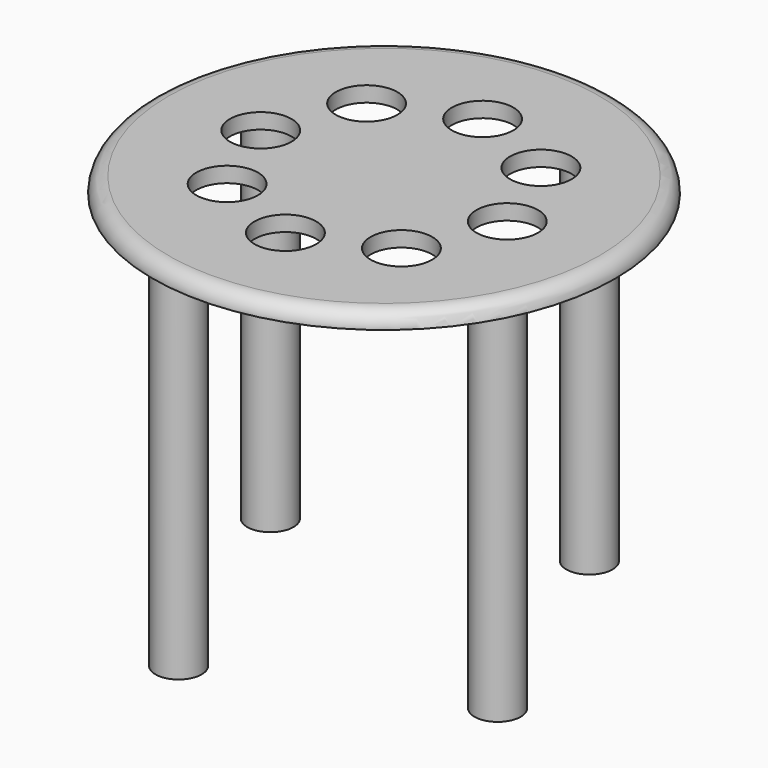
from build123d import *

# Parameters (mm, degrees)
F0_R     = 75
F0_R_2   = 10
F1_DEPTH = 5
F2_R     = 4.99999
F3_R     = 7.5
F4_DEPTH = 120


# Not quite as in the source:
# - a fillet or chamfer is up to 0.001 mm smaller than in the source, because OpenCascade refuses the exact size


with BuildPart() as f1:
    # F0 (on Top) → F1 (new body)
    with BuildSketch(Plane.XY):
        Circle(F0_R)
        with Locations((-28.2842712475, -28.2842712475)):
            Circle(F0_R_2, mode=Mode.SUBTRACT)
        with Locations((0, -40)):
            Circle(F0_R_2, mode=Mode.SUBTRACT)
        with Locations((28.2842712475, -28.2842712475)):
            Circle(F0_R_2, mode=Mode.SUBTRACT)
        with Locations((-40, 0)):
            Circle(F0_R_2, mode=Mode.SUBTRACT)
        with Locations((-28.2842712475, 28.2842712475)):
            Circle(F0_R_2, mode=Mode.SUBTRACT)
        with Locations((28.2842712475, 28.2842712475)):
            Circle(F0_R_2, mode=Mode.SUBTRACT)
        with Locations((40, 0)):
            Circle(F0_R_2, mode=Mode.SUBTRACT)
        with Locations((0, 40)):
            Circle(F0_R_2, mode=Mode.SUBTRACT)
    extrude(amount=F1_DEPTH)

    # F2 (radius 5 in the source; OpenCascade refuses exactly that, so slightly less here)
    f2_edges = [f1.edges().sort_by_distance(p)[0] for p in [
        (-75, 0, 5),
    ]]
    fillet(f2_edges, radius=F2_R)

    # F3 (on face) → F4 (join)
    with BuildSketch(Plane(origin=(0, 0, 0), x_dir=(1, 0, 0), z_dir=(0, 0, -1))):
        with Locations((-22.6591762283, 55)):
            Circle(F3_R)
        with Locations((-55, -22.6591762283)):
            Circle(F3_R)
        with Locations((22.6591762283, -55)):
            Circle(F3_R)
        with Locations((55, 22.6591762283)):
            Circle(F3_R)
    extrude(amount=F4_DEPTH)


solid = f1.part
